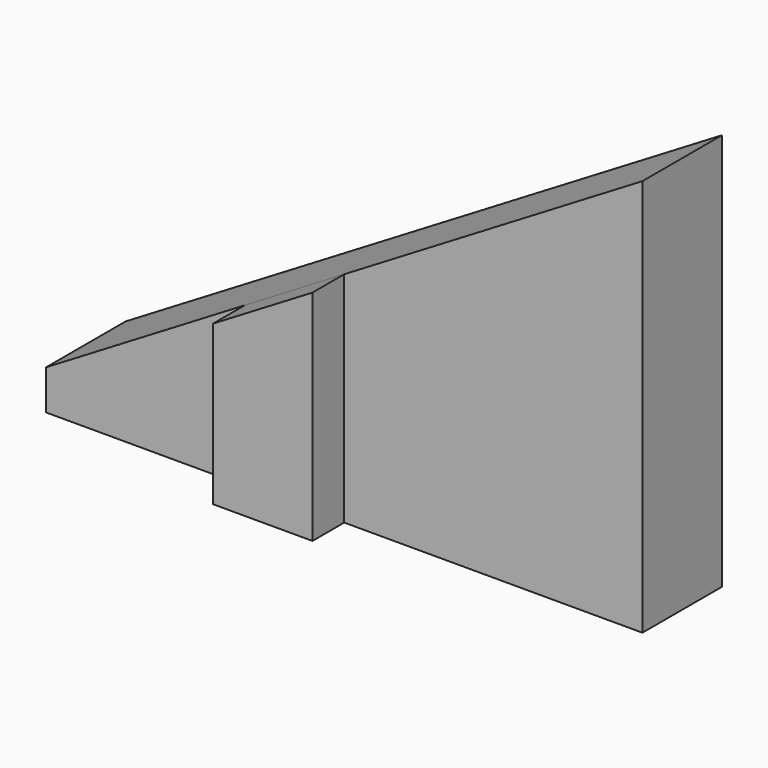
from build123d import *

# Parameters (mm, degrees)
F0_W     = 7620
F0_H     = 5080
F1_DEPTH = 1270
F2_SIZE2 = 7619.99999
F2_SIZE  = 4571.99999
F4_DEPTH = 508


# Not quite as in the source:
# - a fillet or chamfer is up to 0.001 mm smaller than in the source, because OpenCascade refuses the exact size
# - ends of sketch curves that miss each other by under 0.0002 mm in the source are joined


with BuildPart() as f1:
    # F0 (on Front) → F1 (new body)
    with BuildSketch(Plane.XZ):
        Rectangle(F0_W, F0_H)
    extrude(amount=F1_DEPTH)

    # F2 (size 4572 and 7620 in the source; OpenCascade refuses exactly that, so slightly less here)
    f2_edges = [f1.edges().sort_by_distance(p)[0] for p in [
        (-3810, -635, 2540),
    ]]
    f2_side = f1.faces().sort_by_distance((-3810, -635, 0))[0]
    chamfer(f2_edges, length=F2_SIZE, length2=F2_SIZE2, reference=f2_side)

    # F3 (on face) → F4 (join)
    with BuildSketch(Plane.XZ.offset(1270)):
        Polygon((-1270, -508), (-1270, -2540), (0, -2540), (0, 254), align=None)
    extrude(amount=F4_DEPTH)


solid = f1.part
